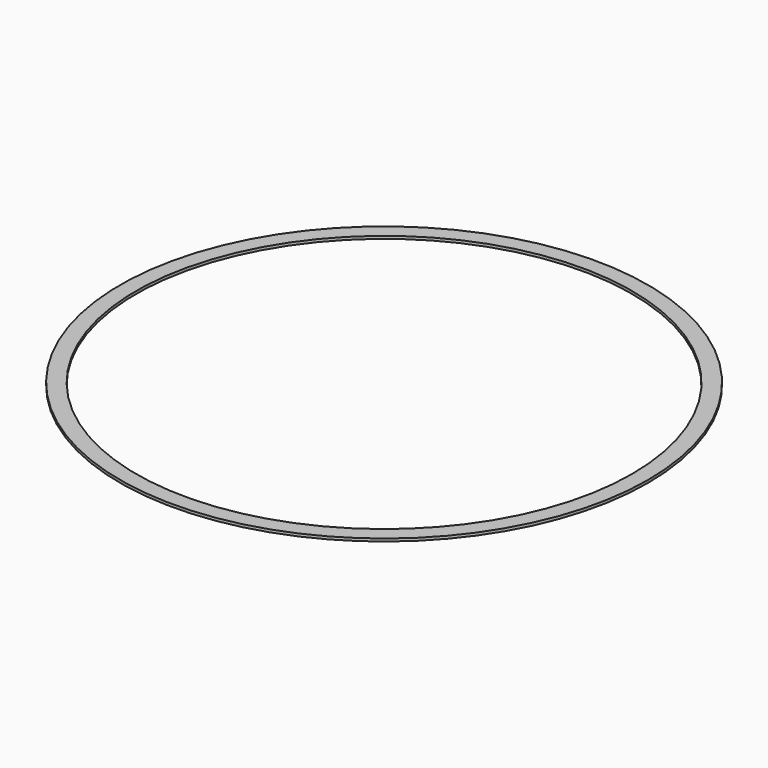
from build123d import *

# Parameters (mm, degrees)
F0_R     = 418.17671
F0_R_2   = 392.77671
F1_DEPTH = 4.2333333333


# Not quite as in the source:
# - a length typed as a fraction of an inch, garbled in the dataset ("3 / 203.2 mm" for 3/8 in), is restored


with BuildPart() as f1:
    # F0 (on Top) → F1 (new body)
    with BuildSketch(Plane.XY):
        Circle(F0_R)
        Circle(F0_R_2, mode=Mode.SUBTRACT)
    extrude(amount=F1_DEPTH)


solid = f1.part
